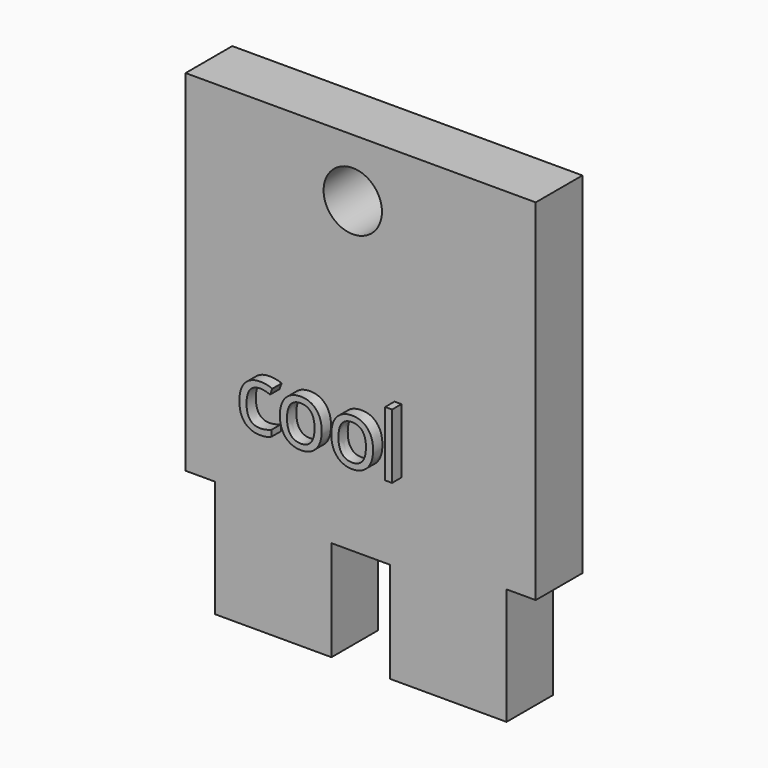
from build123d import *

# Parameters (mm, degrees)
F0_W         = 38.1
F0_H         = 50.8
F1_DEPTH     = 6.35
F2_R         = 3.175
F3_DEPTH     = 6.351
F4_W         = 3.175
F4_H         = 12.7
F5_DEPTH     = 6.351
F7_W         = 6.35
F7_H         = 12.7
F8_DEPTH     = 6.351
F9_TEXT_SIZE = 9.255422096
F10_DEPTH    = 1.27


# Not quite as in the source:
# - Text() gives the source's letters only with a copy of the font that has no kerning and outlines rounded to 1/6400 em; it was checked with that copy


with BuildPart() as f1:
    # F0 (on Front) → F1 (new body)
    with BuildSketch(Plane.XZ):
        with Locations((0.8583124727, 16.0993553412)):
            Rectangle(F0_W, F0_H)
    extrude(amount=F1_DEPTH)

    # F2 (on face) → F3 (cut, through all)
    with BuildSketch(Plane.XZ.offset(6.35)):
        with Locations((0, 35.1493553412)):
            Circle(F2_R)
    extrude(amount=-F3_DEPTH, mode=Mode.SUBTRACT)

    # F4 (on face) → F5 (cut, through all)
    with BuildSketch(Plane.XZ.offset(6.35)):
        with Locations((-16.6041875273, -2.9506446588)):
            Rectangle(F4_W, F4_H)
        with Locations((18.3208124727, -2.9506446588)):
            Rectangle(F4_W, F4_H)
    extrude(amount=-F5_DEPTH, mode=Mode.SUBTRACT)

    # F7 (on face) → F8 (cut, through all)
    with BuildSketch(Plane.XZ.offset(6.35)):
        with Locations((0.8583124727, -4.7194904864)):
            Rectangle(F7_W, F7_H)
    extrude(amount=-F8_DEPTH, mode=Mode.SUBTRACT)

    # F9 (on face) → F10 (join)
    with BuildSketch(Plane.XZ.offset(6.35)):
        with Locations((-11.8416875273, 10.3878446569)):
            Text('cool', F9_TEXT_SIZE, font='Open Sans', text_align=(TextAlign.LEFT, TextAlign.BOTTOM))
    extrude(amount=F10_DEPTH)


solid = f1.part
